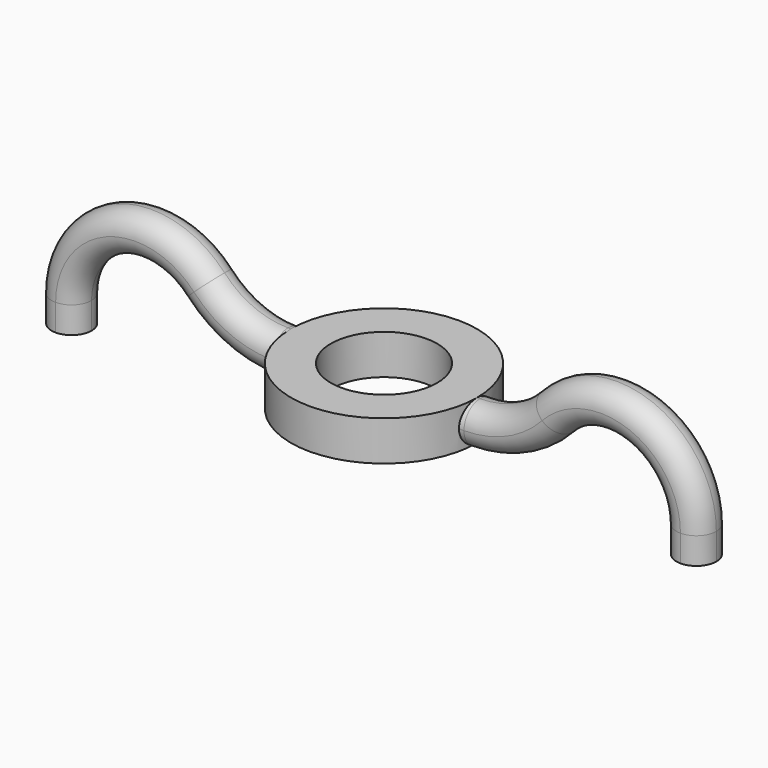
from build123d import *

# Parameters (mm, degrees)
F1_DEPTH = 1.5
F2_R     = 1.49999
F3_R     = 7
F4_DEPTH = 3
F5_R     = 4
F6_DEPTH = 25


# Not quite as in the source:
# - a fillet or chamfer is up to 0.001 mm smaller than in the source, because OpenCascade refuses the exact size


with BuildPart() as f1:
    # F0 (on Front) → F1 (new body, symmetric)
    with BuildSketch(Plane.XZ):
        with BuildLine():
            ThreePointArc((-11.990991839, 5.0892857143), (-20.2324383609, 6.9845386823), (-25, 0))
            Line((-25, 0), (-25, -2))
            Line((-25, -2), (-22, -2))
            Line((-22, -2), (-22, 0))
            ThreePointArc((-22, 0), (-19.1394630165, 4.1907232094), (-14.1945951034, 3.0535714286))
            ThreePointArc((-14.1945951034, 3.0535714286), (-11.0249907967, 0.7968088775), (-7.2165180994, 0))
            Line((-7.2165180994, 0), (0, 0))
            Line((0, 0), (7.2165180994, 0))
            ThreePointArc((7.2165180994, 0), (11.0249907967, 0.7968088775), (14.1945951034, 3.0535714286))
            ThreePointArc((14.1945951034, 3.0535714286), (19.1394630165, 4.1907232094), (22, 0))
            Line((22, 0), (22, -2))
            Line((22, -2), (25, -2))
            Line((25, -2), (25, 0))
            ThreePointArc((25, 0), (20.2324383609, 6.9845386823), (11.990991839, 5.0892857143))
            ThreePointArc((11.990991839, 5.0892857143), (9.822315208, 3.5451850215), (7.2165180994, 3))
            Line((7.2165180994, 3), (0, 3))
            Line((0, 3), (-7.2165180994, 3))
            ThreePointArc((-7.2165180994, 3), (-9.822315208, 3.5451850215), (-11.990991839, 5.0892857143))
        make_face()
    extrude(amount=F1_DEPTH, both=True)

    # F2 (radius 1.5 in the source; OpenCascade refuses exactly that, so slightly less here)
    f2_edges = [f1.edges().sort_by_distance(p)[0] for p in [
        (-20.232438, -1.5, 6.984539),
        (-19.139463, -1.5, 4.190723),
        (-20.232438, 1.5, 6.984539),
        (-19.139463, 1.5, 4.190723),
    ]]
    fillet(f2_edges, radius=F2_R)

    # F3 (on Top) → F4 (join)
    with BuildSketch(Plane.XY):
        Circle(F3_R)
    extrude(amount=F4_DEPTH)

    # F5 (on face) → F6 (cut)
    with BuildSketch(Plane.XY.offset(3)):
        Circle(F5_R)
    extrude(amount=-F6_DEPTH, mode=Mode.SUBTRACT)


solid = f1.part
